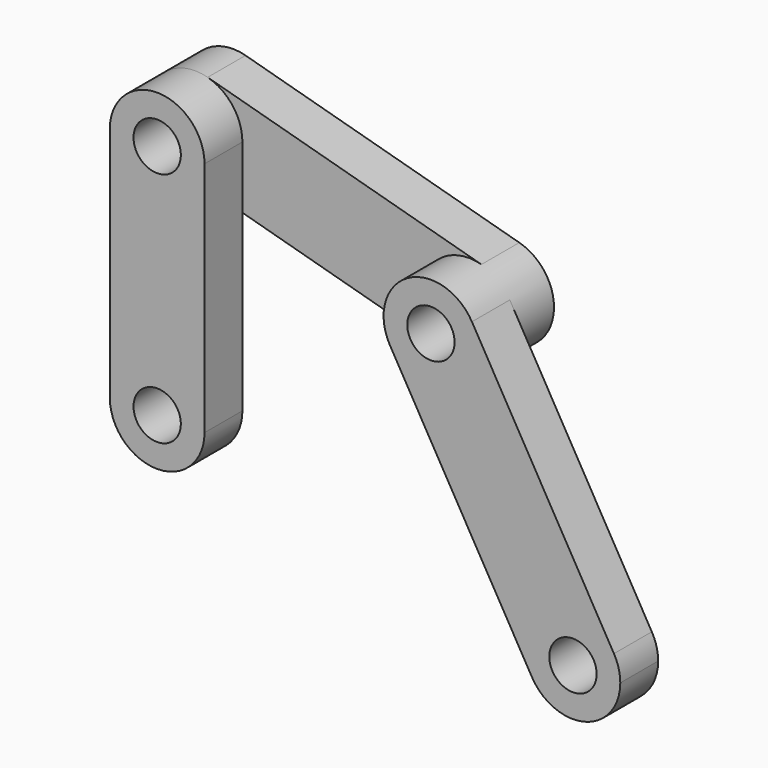
from build123d import *
from build123d import SkipClean  # not in build123d's __all__

# Parameters (mm, degrees)
F0_R     = 6.35
F1_DEPTH = 12.7
F2_R     = 6.35
F3_DEPTH = 12.7
F4_R     = 6.35
F5_DEPTH = 12.7


# Not quite as in the source:
# - after a boolean that leaves OpenCascade's solid faulty, fix() repairs it


with BuildPart() as f1:
    # F0 (on Front) → F1 (new body)
    with BuildSketch(Plane.XZ):
        with BuildLine():
            ThreePointArc((-12.7, 0), (0, -12.7), (12.7, 0))
            ThreePointArc((12.7, 0), (0, 12.7), (-12.7, 0))
        make_face()
        Circle(F0_R, mode=Mode.SUBTRACT)
        with BuildLine():
            Line((12.7, -63.5), (12.7, 0))
            ThreePointArc((12.7, 0), (0, -12.7), (-12.7, 0))
            Line((-12.7, 0), (-12.7, -63.5))
            ThreePointArc((-12.7, -63.5), (0, -50.8), (12.7, -63.5))
        make_face()
        with BuildLine():
            ThreePointArc((-12.7, -63.5), (0, -76.2), (12.7, -63.5))
            ThreePointArc((12.7, -63.5), (0, -50.8), (-12.7, -63.5))
        make_face()
        with Locations((0, -63.5)):
            Circle(F0_R, mode=Mode.SUBTRACT)
    extrude(amount=F1_DEPTH)

    # F2 (on face) → F3 (join)
    with BuildSketch(Plane(origin=(0, 0, 0), x_dir=(-1, 0, 0), z_dir=(0, 1, 0))):
        with BuildLine():
            ThreePointArc((3.3866666667, -12.2401180096), (10.1069448071, -7.6902318994), (12.7, 0))
            ThreePointArc((12.7, 0), (7.6902318994, 10.1069448071), (-3.3866666667, 12.2401180096))
            ThreePointArc((-3.3866666667, 12.2401180096), (-12.2401180096, -3.3866666667), (3.3866666667, -12.2401180096))
        make_face()
        Circle(F2_R, mode=Mode.SUBTRACT)
        with BuildLine():
            ThreePointArc((3.3866666667, -12.2401180096), (-12.2401180096, -3.3866666667), (-3.3866666667, 12.2401180096))
            Line((-3.3866666667, 12.2401180096), (-76.8273747243, -8.0798819904))
            ThreePointArc((-76.8273747243, -8.0798819904), (-65.7504761582, -10.2130551929), (-60.7407080576, -20.32))
            ThreePointArc((-60.7407080576, -20.32), (-63.3337632505, -28.0102318994), (-70.0540413909, -32.5601180096))
            Line((-70.0540413909, -32.5601180096), (3.3866666667, -12.2401180096))
        make_face()
        with BuildLine():
            ThreePointArc((-60.7407080576, -20.32), (-65.7504761582, -10.2130551929), (-76.8273747243, -8.0798819904))
            ThreePointArc((-76.8273747243, -8.0798819904), (-85.6808260672, -23.7066666667), (-70.0540413909, -32.5601180096))
            ThreePointArc((-70.0540413909, -32.5601180096), (-63.3337632505, -28.0102318994), (-60.7407080576, -20.32))
        make_face()
        with Locations((-73.4407080576, -20.32)):
            Circle(F2_R, mode=Mode.SUBTRACT)
    with SkipClean():  # cleaning this boolean's faces spoils the solid; the shape is the same uncleaned
        extrude(amount=F3_DEPTH)

    # F4 (on face) → F5 (join)
    with BuildSketch(Plane.XZ):
        with BuildLine():
            ThreePointArc((62.4421854295, -26.67), (76.7277099304, -32.5872579939), (86.1407080576, -20.32))
            ThreePointArc((86.1407080576, -20.32), (85.7079660515, -17.0329981272), (84.4392306857, -13.97))
            ThreePointArc((84.4392306857, -13.97), (67.0907080576, -9.3214773719), (62.4421854295, -26.67))
        make_face()
        with Locations((73.4407080576, -20.32)):
            Circle(F4_R, mode=Mode.SUBTRACT)
        with BuildLine():
            ThreePointArc((84.4392306857, -13.97), (85.7079660515, -17.0329981272), (86.1407080576, -20.32))
            ThreePointArc((86.1407080576, -20.32), (76.7277099304, -32.5872579939), (62.4421854295, -26.67))
            Line((62.4421854295, -26.67), (100.5421854295, -92.6611357684))
            ThreePointArc((100.5421854295, -92.6611357684), (105.1907080576, -75.3126131403), (122.5392306857, -79.9611357684))
            Line((122.5392306857, -79.9611357684), (84.4392306857, -13.97))
        make_face()
        with BuildLine():
            ThreePointArc((124.2407080576, -86.3111357684), (123.8079660515, -83.0241338956), (122.5392306857, -79.9611357684))
            ThreePointArc((122.5392306857, -79.9611357684), (105.1907080576, -75.3126131403), (100.5421854295, -92.6611357684))
            ThreePointArc((100.5421854295, -92.6611357684), (114.8277099304, -98.5783937622), (124.2407080576, -86.3111357684))
        make_face()
        with Locations((111.5407080576, -86.3111357684)):
            Circle(F4_R, mode=Mode.SUBTRACT)
    extrude(amount=F5_DEPTH)

    add(f1.part.fix(), mode=Mode.REPLACE)


solid = f1.part
